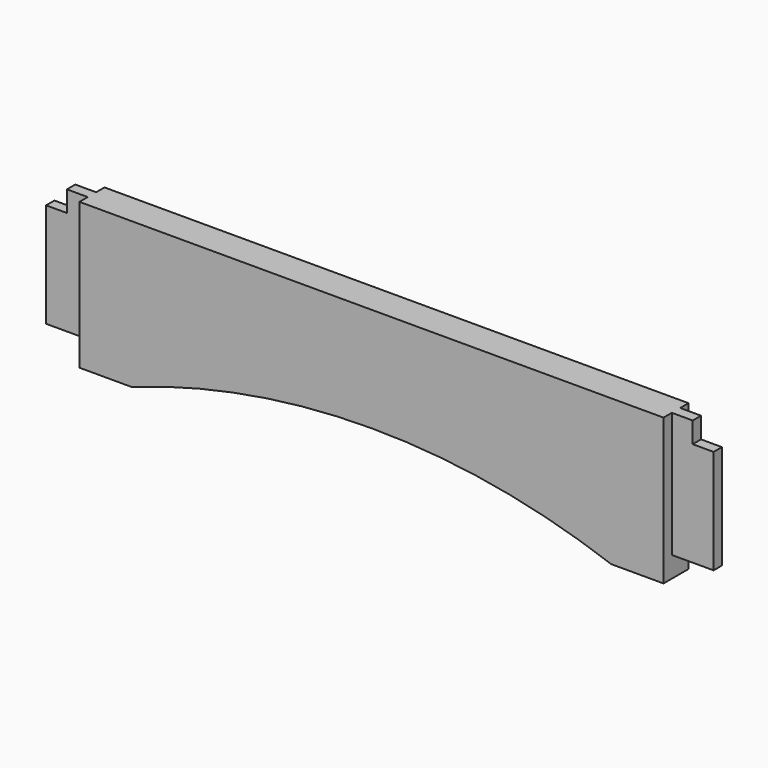
from build123d import *

# Parameters (mm, degrees)
F0_W     = 355.6
F0_H     = 88.9
F1_DEPTH = 9.525
F3_DEPTH = 3.175
F5_DEPTH = 19.05


# Not quite as in the source:
# - a pattern or mirror of a feature is missing from the dataset's text; its kind, count and spacing are read off the source's solid


with BuildPart() as f1:
    # F0 (on Front) → F1 (new body, symmetric)
    with BuildSketch(Plane.XZ):
        Rectangle(F0_W, F0_H)
    extrude(amount=F1_DEPTH, both=True)

    # F2 (on Front) → F3 (join, symmetric)
    with BuildSketch(Plane.XZ):
        Polygon((-177.8, -31.75), (-177.8, 44.45), (-190.5, 44.45), (-190.5, 31.75), (-203.2, 31.75), (-203.2, -31.75), align=None)
    f3 = extrude(amount=F3_DEPTH, both=True)

    # F3_copies: F3 across plane
    add(f3.mirror(Plane(origin=(0, 0, 0), x_dir=(0, 0, 1), z_dir=(1, 0, 0))))

    # F4 (on face) → F5 (cut, through all)
    with BuildSketch(Plane.XZ.offset(9.525)):
        with BuildLine():
            ThreePointArc((146.05, -44.45), (0, -19.05), (-146.05, -44.45))
            Line((-146.05, -44.45), (146.05, -44.45))
        make_face()
    extrude(amount=-F5_DEPTH, mode=Mode.SUBTRACT)


solid = f1.part
